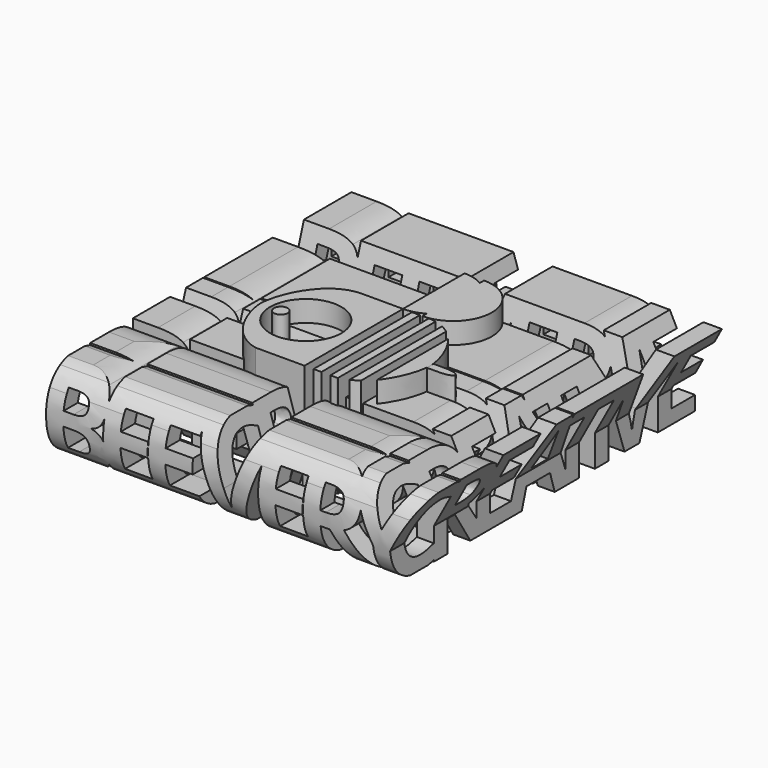
from build123d import *

# Parameters (mm, degrees)
F0_W     = 0.4192708333
F0_H     = 3.4461805556
F0_H_2   = 3.4722222222
F1_DEPTH = 200
F2_W     = 0.579117015
F2_H     = 3.4982638889
F3_DEPTH = 200
F6_DEPTH = 25
F5_W     = 1.9421083595
F5_H     = 30.1811452955
F5_R     = 8.7336650025
F5_R_2   = 1.6761545088


# Not quite as in the source:
# - a feature of the source that left no trace in its solid (it failed there, or was rolled back) is left out
# - a feature names something its author has since deleted; it is built from what else it names


with BuildPart() as f1:
    # F0 (on Front) → F1 (new body)
    with BuildSketch(Plane.XZ):
        with BuildLine():
            Line((8.6675347222, 19.8307291667), (2.4956597222, 19.8307291667))
            Line((2.4956597222, 19.8307291667), (2.4956597222, 0))
            Line((2.4956597222, 0), (9.9131944444, 0))
            add(Edge.make_bspline(
                [(15.2387152778, 1.5190972222), (13.2769097222, 0), (9.9131944444, 0)],
                knots=[0, 0, 0, 1, 1, 1], degree=2))
            add(Edge.make_bspline(
                [(16.4956597222, 2.9277045824), (16.024595477, 2.1276327747), (15.2387152778, 1.5190972222)],
                knots=[0.5994097392, 0.5994097392, 0.5994097392, 1, 1, 1], degree=2))
            Line((16.4956597222, 2.9277045824), (16.4956597222, 8.6243749651))
            add(Edge.make_bspline(
                [(16.3650173611, 8.8172743056), (16.4331135713, 8.7233545974), (16.4956597222, 8.6243749651)],
                knots=[0, 0, 0, 0.0815032043, 0.0815032043, 0.0815032043], degree=2))
            add(Edge.make_bspline(
                [(13.6458333333, 10.390625), (15.5295138889, 9.9696180556), (16.3650173611, 8.8172743056)],
                knots=[0, 0, 0, 1, 1, 1], degree=2))
            Line((13.6458333333, 10.390625), (13.6458333333, 10.5251736111))
            add(Edge.make_bspline(
                [(15.8637152778, 11.89453125), (15.0303819444, 10.7552083333), (13.6458333333, 10.5251736111)],
                knots=[0, 0, 0, 1, 1, 1], degree=2))
            add(Edge.make_bspline(
                [(16.4956597222, 13.2184769116), (16.2873852443, 12.4737675324), (15.8637152778, 11.89453125)],
                knots=[0.4915960401, 0.4915960401, 0.4915960401, 1, 1, 1], degree=2))
            Line((16.4956597222, 13.2184769116), (16.4956597222, 16.3653214947))
            add(Edge.make_bspline(
                [(14.7916666667, 18.6306423611), (16.0775950191, 17.8207125446), (16.4956597222, 16.3653214947)],
                knots=[0, 0, 0, 0.6748926934, 0.6748926934, 0.6748926934], degree=2))
            add(Edge.make_bspline(
                [(8.6675347222, 19.8307291667), (12.8862847222, 19.8307291667), (14.7916666667, 18.6306423611)],
                knots=[0, 0, 0, 1, 1, 1], degree=2))
        make_face()
        with BuildLine():
            Line((6.7013888889, 3.4722222222), (6.7013888889, 8.6414930556))
            Line((6.7013888889, 8.6414930556), (9.3055555556, 8.6414930556))
            add(Edge.make_bspline(
                [(12.8298611111, 6.171875), (12.8298611111, 8.6414930556), (9.3055555556, 8.6414930556)],
                knots=[0, 0, 0, 1, 1, 1], degree=2))
            add(Edge.make_bspline(
                [(12.0030381944, 4.1362847222), (12.8298611111, 4.8003472222), (12.8298611111, 6.171875)],
                knots=[0, 0, 0, 1, 1, 1], degree=2))
            add(Edge.make_bspline(
                [(9.4401041667, 3.4722222222), (11.1762152778, 3.4722222222), (12.0030381944, 4.1362847222)],
                knots=[0, 0, 0, 1, 1, 1], degree=2))
            Line((9.4401041667, 3.4722222222), (6.7013888889, 3.4722222222))
        make_face(mode=Mode.SUBTRACT)
        with BuildLine():
            Line((9.140625, 11.9748263889), (6.7013888889, 11.9748263889))
            Line((6.7013888889, 11.9748263889), (6.7013888889, 16.3845486111))
            Line((6.7013888889, 16.3845486111), (8.9105902778, 16.3845486111))
            add(Edge.make_bspline(
                [(11.5494791667, 15.8897569444), (10.7161458333, 16.3845486111), (8.9105902778, 16.3845486111)],
                knots=[0, 0, 0, 1, 1, 1], degree=2))
            add(Edge.make_bspline(
                [(12.3828125, 14.2534722222), (12.3828125, 15.3949652778), (11.5494791667, 15.8897569444)],
                knots=[0, 0, 0, 1, 1, 1], degree=2))
            add(Edge.make_bspline(
                [(11.6167534722, 12.5043402778), (12.3828125, 13.0338541667), (12.3828125, 14.2534722222)],
                knots=[0, 0, 0, 1, 1, 1], degree=2))
            add(Edge.make_bspline(
                [(9.140625, 11.9748263889), (10.8506944444, 11.9748263889), (11.6167534722, 12.5043402778)],
                knots=[0, 0, 0, 1, 1, 1], degree=2))
        make_face(mode=Mode.SUBTRACT)
        with BuildLine():
            Line((16.4956597222, 19.8307291667), (16.4956597222, 16.3653214947))
            add(Edge.make_bspline(
                [(16.4956597222, 16.3653214947), (16.6970486111, 15.6642348346), (16.6970486111, 14.8133680556)],
                knots=[0.6748926934, 0.6748926934, 0.6748926934, 1, 1, 1], degree=2))
            add(Edge.make_bspline(
                [(16.6970486111, 14.8133680556), (16.6970486111, 13.9385660744), (16.4956597222, 13.2184769116)],
                knots=[0, 0, 0, 0.4915960401, 0.4915960401, 0.4915960401], degree=2))
            Line((16.4956597222, 13.2184769116), (16.4956597222, 8.6243749651))
            add(Edge.make_bspline(
                [(16.4956597222, 8.6243749651), (17.2005208333, 7.5089283285), (17.2005208333, 5.7508680556)],
                knots=[0.0815032043, 0.0815032043, 0.0815032043, 1, 1, 1], degree=2))
            add(Edge.make_bspline(
                [(17.2005208333, 5.7508680556), (17.2005208333, 4.1248650739), (16.4956597222, 2.9277045824)],
                knots=[0, 0, 0, 0.5994097392, 0.5994097392, 0.5994097392], degree=2))
            Line((16.4956597222, 2.9277045824), (16.4956597222, 0))
            Line((16.4956597222, 0), (27.4956597222, 0))
            Line((27.4956597222, 0), (27.4956597222, 3.4722222222))
            Line((27.4956597222, 3.4722222222), (20.7013888889, 3.4722222222))
            Line((20.7013888889, 3.4722222222), (20.7013888889, 8.5850694444))
            Line((20.7013888889, 8.5850694444), (27.4157986111, 8.5850694444))
            Line((27.4157986111, 8.5850694444), (27.4157986111, 12.03125))
            Line((27.4157986111, 12.03125), (20.7013888889, 12.03125))
            Line((20.7013888889, 12.03125), (20.7013888889, 16.3845486111))
            Line((20.7013888889, 16.3845486111), (27.4956597222, 16.3845486111))
            Line((27.4956597222, 16.3845486111), (27.4956597222, 19.8307291667))
            Line((27.4956597222, 19.8307291667), (16.4956597222, 19.8307291667))
        make_face()
        with BuildLine():
            Line((16.4956597222, 8.6243749651), (16.4956597222, 2.9277045824))
            add(Edge.make_bspline(
                [(17.2005208333, 5.7508680556), (17.2005208333, 4.1248650739), (16.4956597222, 2.9277045824)],
                knots=[0, 0, 0, 0.5994097392, 0.5994097392, 0.5994097392], degree=2))
            add(Edge.make_bspline(
                [(16.4956597222, 8.6243749651), (17.2005208333, 7.5089283285), (17.2005208333, 5.7508680556)],
                knots=[0.0815032043, 0.0815032043, 0.0815032043, 1, 1, 1], degree=2))
        make_face()
        with BuildLine():
            add(Edge.make_bspline(
                [(16.4956597222, 16.3653214947), (16.6970486111, 15.6642348346), (16.6970486111, 14.8133680556)],
                knots=[0.6748926934, 0.6748926934, 0.6748926934, 1, 1, 1], degree=2))
            Line((16.4956597222, 16.3653214947), (16.4956597222, 13.2184769116))
            add(Edge.make_bspline(
                [(16.6970486111, 14.8133680556), (16.6970486111, 13.9385660744), (16.4956597222, 13.2184769116)],
                knots=[0, 0, 0, 0.4915960401, 0.4915960401, 0.4915960401], degree=2))
        make_face()
        Polygon((38, 19.8307291667), (27.9149305556, 19.8307291667), (27.9149305556, 16.3845486111), (27.4956597222, 16.3845486111), (27.4956597222, 3.4722222222), (27.9149305556, 3.4722222222), (27.9149305556, 0), (38.9149305556, 0), (38.9149305556, 3.4722222222), (31.7013888889, 3.4722222222), (31.7013888889, 8.5850694444), (38.4157986111, 8.5850694444), (38.4157986111, 12.03125), (31.7013888889, 12.03125), (31.7013888889, 16.3845486111), (38.9149305556, 16.3845486111), (38.9149305556, 17.13375), align=None)
        with Locations((27.7052951389, 18.1076388889)):
            Rectangle(F0_W, F0_H)
        with Locations((27.7052951389, 1.7361111111)):
            Rectangle(F0_W, F0_H_2)
        with BuildLine():
            Line((42.2447916667, 19.8307291667), (38.9149305556, 19.8307291667))
            Line((38.9149305556, 19.8307291667), (38.9149305556, 17.13375))
            Line((38.9149305556, 17.13375), (44.7274305556, 0))
            Line((44.7274305556, 0), (49.3107638889, 0))
            Line((49.3107638889, 0), (54.4956597222, 15.2542106005))
            Line((54.4956597222, 15.2542106005), (54.4956597222, 19.8307291667))
            Line((54.4956597222, 19.8307291667), (51.8064236111, 19.8307291667))
            Line((51.8064236111, 19.8307291667), (48.0520833333, 8.0295138889))
            add(Edge.make_bspline(
                [(47.0321180556, 3.6631944444), (47.1840277778, 4.9088541667), (48.0520833333, 8.0295138889)],
                knots=[0, 0, 0, 1, 1, 1], degree=2))
            add(Edge.make_bspline(
                [(46.6197916667, 5.5946180556), (46.9539930556, 4.2057291667), (47.0321180556, 3.6631944444)],
                knots=[0, 0, 0, 1, 1, 1], degree=2))
            add(Edge.make_bspline(
                [(45.9774305556, 8.0295138889), (46.2855902778, 6.9835069444), (46.6197916667, 5.5946180556)],
                knots=[0, 0, 0, 1, 1, 1], degree=2))
            Line((45.9774305556, 8.0295138889), (42.2447916667, 19.8307291667))
        make_face()
        Polygon((38.9149305556, 19.8307291667), (38, 19.8307291667), (38.9149305556, 17.13375), align=None)
        Polygon((54.4956597222, 19.8307291667), (54.4956597222, 15.2542106005), (56.0512152778, 19.8307291667), align=None)
        Polygon((56.0512152778, 19.8307291667), (54.4956597222, 15.2542106005), (54.4956597222, 0), (65.4956597222, 0), (65.4956597222, 3.4722222222), (58.7013888889, 3.4722222222), (58.7013888889, 8.5850694444), (65.4157986111, 8.5850694444), (65.4157986111, 12.03125), (58.7013888889, 12.03125), (58.7013888889, 16.3845486111), (65.4956597222, 16.3845486111), (65.4956597222, 19.8307291667), align=None)
        with Locations((65.7052951389, 18.1076388889)):
            Rectangle(F0_W, F0_H)
        with BuildLine():
            Line((71.2725694444, 19.8307291667), (65.9149305556, 19.8307291667))
            Line((65.9149305556, 19.8307291667), (65.9149305556, 16.3845486111))
            Line((65.9149305556, 16.3845486111), (65.4956597222, 16.3845486111))
            Line((65.4956597222, 16.3845486111), (65.4956597222, 3.4722222222))
            Line((65.4956597222, 3.4722222222), (65.9149305556, 3.4722222222))
            Line((65.9149305556, 3.4722222222), (65.9149305556, 0))
            Line((65.9149305556, 0), (69.7013888889, 0))
            Line((69.7013888889, 0), (69.7013888889, 7.6085069444))
            Line((69.7013888889, 7.6085069444), (71.9366319444, 7.6085069444))
            Line((71.9366319444, 7.6085069444), (76.671875, 0))
            Line((76.671875, 0), (81.3376736111, 0))
            add(Edge.make_bspline(
                [(75.5043402778, 8.6414930556), (79.9835069444, 1.953125), (81.3376736111, 0)],
                knots=[0, 0, 0, 1, 1, 1], degree=2))
            add(Edge.make_bspline(
                [(78.2322048611, 10.7769097222), (77.2708333333, 9.4140625), (75.5043402778, 8.6414930556)],
                knots=[0, 0, 0, 1, 1, 1], degree=2))
            add(Edge.make_bspline(
                [(79.1935757147, 13.8859595975), (79.1927713045, 12.138615651), (78.2322048611, 10.7769097222)],
                knots=[0.0008374332, 0.0008374332, 0.0008374332, 1, 1, 1], degree=2))
            Line((79.1935757147, 13.8859595975), (76.5480062099, 18.8106278972))
            add(Edge.make_bspline(
                [(71.2725694444, 19.8307291667), (74.640758574, 19.8307291667), (76.5480062099, 18.8106278972)],
                knots=[0, 0, 0, 0.8326510466, 0.8326510466, 0.8326510466], degree=2))
        make_face()
        with BuildLine():
            Line((71.0555555556, 11.0286458333), (69.7013888889, 11.0286458333))
            Line((69.7013888889, 11.0286458333), (69.7013888889, 16.3845486111))
            Line((69.7013888889, 16.3845486111), (70.9774305556, 16.3845486111))
            add(Edge.make_bspline(
                [(73.9787326389, 15.7877604167), (73.0086805556, 16.3845486111), (70.9774305556, 16.3845486111)],
                knots=[0, 0, 0, 1, 1, 1], degree=2))
            add(Edge.make_bspline(
                [(74.9487847222, 13.7803819444), (74.9487847222, 15.1909722222), (73.9787326389, 15.7877604167)],
                knots=[0, 0, 0, 1, 1, 1], degree=2))
            add(Edge.make_bspline(
                [(74.0004340278, 11.6927083333), (74.9487847222, 12.3567708333), (74.9487847222, 13.7803819444)],
                knots=[0, 0, 0, 1, 1, 1], degree=2))
            add(Edge.make_bspline(
                [(71.0555555556, 11.0286458333), (73.0520833333, 11.0286458333), (74.0004340278, 11.6927083333)],
                knots=[0, 0, 0, 1, 1, 1], degree=2))
        make_face(mode=Mode.SUBTRACT)
        with Locations((65.7052951389, 1.7361111111)):
            Rectangle(F0_W, F0_H_2)
        with BuildLine():
            add(Edge.make_bspline(
                [(76.5480062099, 18.8106278972), (76.9313311298, 18.6056045799), (77.2556423611, 18.359375)],
                knots=[0.8326510466, 0.8326510466, 0.8326510466, 1, 1, 1], degree=2))
            Line((76.5480062099, 18.8106278972), (79.1935757147, 13.8859595975))
            add(Edge.make_bspline(
                [(79.1935763889, 13.8888888889), (79.1935763889, 13.8874241078), (79.1935757147, 13.8859595975)],
                knots=[0, 0, 0, 0.0008374332, 0.0008374332, 0.0008374332], degree=2))
            add(Edge.make_bspline(
                [(77.2556423611, 18.359375), (79.1935763889, 16.8880208333), (79.1935763889, 13.8888888889)],
                knots=[0, 0, 0, 1, 1, 1], degree=2))
        make_face()
        with BuildLine():
            Line((76, 19.8307291667), (76.5480062099, 18.8106278972))
            add(Edge.make_bspline(
                [(76.5480062099, 18.8106278972), (76.9313311298, 18.6056045799), (77.2556423611, 18.359375)],
                knots=[0.8326510466, 0.8326510466, 0.8326510466, 1, 1, 1], degree=2))
            add(Edge.make_bspline(
                [(77.2556423611, 18.359375), (79.1935763889, 16.8880208333), (79.1935763889, 13.8888888889)],
                knots=[0, 0, 0, 1, 1, 1], degree=2))
            add(Edge.make_bspline(
                [(79.1935763889, 13.8888888889), (79.1935763889, 13.8874241078), (79.1935757147, 13.8859595975)],
                knots=[0, 0, 0, 0.0008374332, 0.0008374332, 0.0008374332], degree=2))
            Line((79.1935757147, 13.8859595975), (82.5798611111, 7.5824652778))
            Line((82.5798611111, 7.5824652778), (82.5798611111, 0))
            Line((82.5798611111, 0), (86.7552083333, 0))
            Line((86.7552083333, 0), (86.7552083333, 7.7170138889))
            Line((86.7552083333, 7.7170138889), (93.3350694444, 19.8307291667))
            Line((93.3350694444, 19.8307291667), (88.8038194444, 19.8307291667))
            Line((88.8038194444, 19.8307291667), (84.6675347222, 11.6666666667))
            Line((84.6675347222, 11.6666666667), (80.5572916667, 19.8307291667))
            Line((80.5572916667, 19.8307291667), (76, 19.8307291667))
        make_face()
    extrude(amount=-F1_DEPTH)


with BuildPart() as f3:
    # F2 (on Right) → F3 (new body)
    with BuildSketch(Plane.YZ):
        with BuildLine():
            add(Edge.make_bspline(
                [(10.9201388889, 16.6145833333), (8.5460069444, 16.6145833333), (7.2439236111, 14.8307291667)],
                knots=[0, 0, 0, 1, 1, 1], degree=2))
            add(Edge.make_bspline(
                [(13.1293402778, 16.2217881944), (12.0052083333, 16.6145833333), (10.9201388889, 16.6145833333)],
                knots=[0, 0, 0, 1, 1, 1], degree=2))
            add(Edge.make_bspline(
                [(15.1430216173, 15.405273706), (14.139687044, 15.8687519692), (13.1293402778, 16.2217881944)],
                knots=[0.1012204829, 0.1012204829, 0.1012204829, 1, 1, 1], degree=2))
            Line((15.1430216173, 15.405273706), (15.1430216173, 19.3729401919))
            add(Edge.make_bspline(
                [(10.9201388889, 20.1128472222), (13.023512731, 20.1128472222), (15.1430216173, 19.3729401919)],
                knots=[0, 0, 0, 0.7287478695, 0.7287478695, 0.7287478695], degree=2))
            add(Edge.make_bspline(
                [(5.9765625, 18.8736979167), (8.0859375, 20.1128472222), (10.9201388889, 20.1128472222)],
                knots=[0, 0, 0, 1, 1, 1], degree=2))
            add(Edge.make_bspline(
                [(2.7408854167, 15.3081597222), (3.8671875, 17.6345486111), (5.9765625, 18.8736979167)],
                knots=[0, 0, 0, 1, 1, 1], degree=2))
            add(Edge.make_bspline(
                [(1.6145833333, 9.8871527778), (1.6145833333, 12.9817708333), (2.7408854167, 15.3081597222)],
                knots=[0, 0, 0, 1, 1, 1], degree=2))
            add(Edge.make_bspline(
                [(3.90625, 2.3524305556), (1.6145833333, 4.9782986111), (1.6145833333, 9.8871527778)],
                knots=[0, 0, 0, 1, 1, 1], degree=2))
            add(Edge.make_bspline(
                [(10.5251736111, -0.2734375), (6.1979166667, -0.2734375), (3.90625, 2.3524305556)],
                knots=[0, 0, 0, 1, 1, 1], degree=2))
            add(Edge.make_bspline(
                [(15.1430216173, 0.4333476683), (13.0325989806, -0.2734375), (10.5251736111, -0.2734375)],
                knots=[0.1675636814, 0.1675636814, 0.1675636814, 1, 1, 1], degree=2))
            Line((15.1430216173, 0.4333476683), (15.1430216173, 3.9934341916))
            add(Edge.make_bspline(
                [(10.9201388889, 3.2291666667), (12.708358779, 3.2291666667), (15.1430216173, 3.9934341916)],
                knots=[0, 0, 0, 0.8565610451, 0.8565610451, 0.8565610451], degree=2))
            add(Edge.make_bspline(
                [(5.9418402778, 9.8611111111), (5.9418402778, 3.2291666667), (10.9201388889, 3.2291666667)],
                knots=[0, 0, 0, 1, 1, 1], degree=2))
            add(Edge.make_bspline(
                [(7.2439236111, 14.8307291667), (5.9418402778, 13.046875), (5.9418402778, 9.8611111111)],
                knots=[0, 0, 0, 1, 1, 1], degree=2))
        make_face()
        with BuildLine():
            Line((15.1430216173, 19.3729401919), (15.1430216173, 15.405273706))
            add(Edge.make_bspline(
                [(15.3689236111, 15.2994791667), (15.2560170829, 15.3530768182), (15.1430216173, 15.405273706)],
                knots=[0, 0, 0, 0.1012204829, 0.1012204829, 0.1012204829], degree=2))
            Line((15.3689236111, 15.2994791667), (16.7230902778, 18.7196180556))
            add(Edge.make_bspline(
                [(15.1430216173, 19.3729401919), (15.9319382305, 19.0975344353), (16.7230902778, 18.7196180556)],
                knots=[0.7287478695, 0.7287478695, 0.7287478695, 1, 1, 1], degree=2))
        make_face()
        with BuildLine():
            add(Edge.make_bspline(
                [(15.3689236111, 15.2994791667), (15.2560170829, 15.3530768182), (15.1430216173, 15.405273706)],
                knots=[0, 0, 0, 0.1012204829, 0.1012204829, 0.1012204829], degree=2))
            Line((15.1430216173, 15.405273706), (15.1430216173, 3.9934341916))
            add(Edge.make_bspline(
                [(15.1430216173, 3.9934341916), (15.5507281026, 4.1214177553), (15.9765625, 4.2708333333)],
                knots=[0.8565610451, 0.8565610451, 0.8565610451, 1, 1, 1], degree=2))
            Line((15.9765625, 4.2708333333), (15.9765625, 0.7465277778))
            add(Edge.make_bspline(
                [(15.9765625, 0.7465277778), (15.5678351175, 0.575618641), (15.1430216173, 0.4333476683)],
                knots=[0, 0, 0, 0.1675636814, 0.1675636814, 0.1675636814], degree=2))
            Line((15.1430216173, 0.4333476683), (15.1430216173, 0))
            Line((15.1430216173, 0), (19.348750784, 0))
            Line((19.348750784, 0), (19.348750784, 7.6085069444))
            Line((19.348750784, 7.6085069444), (21.5839938395, 7.6085069444))
            Line((21.5839938395, 7.6085069444), (26.3192368951, 0))
            Line((26.3192368951, 0), (28.2236685377, 0))
            Line((28.2236685377, 0), (28.2236685377, 4.0653140771))
            add(Edge.make_bspline(
                [(25.1517021728, 8.6414930556), (26.9354919994, 5.9779076654), (28.2236685377, 4.0653140771)],
                knots=[0, 0, 0, 0.3982414496, 0.3982414496, 0.3982414496], degree=2))
            add(Edge.make_bspline(
                [(27.8795667562, 10.7769097222), (26.9181952284, 9.4140625), (25.1517021728, 8.6414930556)],
                knots=[0, 0, 0, 1, 1, 1], degree=2))
            add(Edge.make_bspline(
                [(28.2236685377, 11.3337737786), (28.0705970875, 11.0477156998), (27.8795667562, 10.7769097222)],
                knots=[0.8012939579, 0.8012939579, 0.8012939579, 1, 1, 1], degree=2))
            Line((28.2236685377, 11.3337737786), (28.2236685377, 16.7875339058))
            add(Edge.make_bspline(
                [(26.9030042562, 18.359375), (27.7472161778, 17.7184167885), (28.2236685377, 16.7875339058)],
                knots=[0, 0, 0, 0.4356246959, 0.4356246959, 0.4356246959], degree=2))
            add(Edge.make_bspline(
                [(20.9199313395, 19.8307291667), (24.9650702284, 19.8307291667), (26.9030042562, 18.359375)],
                knots=[0, 0, 0, 1, 1, 1], degree=2))
            Line((20.9199313395, 19.8307291667), (15.1430216173, 19.8307291667))
            Line((15.1430216173, 19.8307291667), (15.1430216173, 19.3729401919))
            add(Edge.make_bspline(
                [(15.1430216173, 19.3729401919), (15.9319382305, 19.0975344353), (16.7230902778, 18.7196180556)],
                knots=[0.7287478695, 0.7287478695, 0.7287478695, 1, 1, 1], degree=2))
            Line((16.7230902778, 18.7196180556), (15.3689236111, 15.2994791667))
        make_face()
        with BuildLine():
            Line((20.7029174506, 11.0286458333), (19.348750784, 11.0286458333))
            Line((19.348750784, 11.0286458333), (19.348750784, 16.3845486111))
            Line((19.348750784, 16.3845486111), (20.6247924506, 16.3845486111))
            add(Edge.make_bspline(
                [(23.626094534, 15.7877604167), (22.6560424506, 16.3845486111), (20.6247924506, 16.3845486111)],
                knots=[0, 0, 0, 1, 1, 1], degree=2))
            add(Edge.make_bspline(
                [(24.5961466173, 13.7803819444), (24.5961466173, 15.1909722222), (23.626094534, 15.7877604167)],
                knots=[0, 0, 0, 1, 1, 1], degree=2))
            add(Edge.make_bspline(
                [(23.6477959228, 11.6927083333), (24.5961466173, 12.3567708333), (24.5961466173, 13.7803819444)],
                knots=[0, 0, 0, 1, 1, 1], degree=2))
            add(Edge.make_bspline(
                [(20.7029174506, 11.0286458333), (22.6994452284, 11.0286458333), (23.6477959228, 11.6927083333)],
                knots=[0, 0, 0, 1, 1, 1], degree=2))
        make_face(mode=Mode.SUBTRACT)
        with BuildLine():
            add(Edge.make_bspline(
                [(15.1430216173, 3.9934341916), (15.5507281026, 4.1214177553), (15.9765625, 4.2708333333)],
                knots=[0.8565610451, 0.8565610451, 0.8565610451, 1, 1, 1], degree=2))
            Line((15.1430216173, 3.9934341916), (15.1430216173, 0.4333476683))
            add(Edge.make_bspline(
                [(15.9765625, 0.7465277778), (15.5678351175, 0.575618641), (15.1430216173, 0.4333476683)],
                knots=[0, 0, 0, 0.1675636814, 0.1675636814, 0.1675636814], degree=2))
            Line((15.9765625, 0.7465277778), (15.9765625, 4.2708333333))
        make_face()
        with BuildLine():
            Line((28.2236685377, 19.8307291667), (28.2236685377, 16.7875339058))
            add(Edge.make_bspline(
                [(28.2236685377, 16.7875339058), (28.840938284, 15.5815248919), (28.840938284, 13.8888888889)],
                knots=[0.4356246959, 0.4356246959, 0.4356246959, 1, 1, 1], degree=2))
            add(Edge.make_bspline(
                [(28.840938284, 13.8888888889), (28.840938284, 12.4873200303), (28.2236685377, 11.3337737786)],
                knots=[0, 0, 0, 0.8012939579, 0.8012939579, 0.8012939579], degree=2))
            Line((28.2236685377, 11.3337737786), (28.2236685377, 4.0653140771))
            add(Edge.make_bspline(
                [(28.2236685377, 4.0653140771), (30.1701541359, 1.1753096687), (30.9850355062, 0)],
                knots=[0.3982414496, 0.3982414496, 0.3982414496, 1, 1, 1], degree=2))
            Line((30.9850355062, 0), (37.5626759736, 0))
            Line((37.5626759736, 0), (38.7834027488, 3.4722222222))
            Line((38.7834027488, 3.4722222222), (32.4293977044, 3.4722222222))
            Line((32.4293977044, 3.4722222222), (32.4293977044, 8.5850694444))
            Line((32.4293977044, 8.5850694444), (39.1438074266, 8.5850694444))
            Line((39.1438074266, 8.5850694444), (39.1438074266, 12.03125))
            Line((39.1438074266, 12.03125), (32.4293977044, 12.03125))
            Line((32.4293977044, 12.03125), (32.4293977044, 16.3845486111))
            Line((32.4293977044, 16.3845486111), (39.6429393711, 16.3845486111))
            Line((39.6429393711, 16.3845486111), (39.6429393711, 19.8307291667))
            Line((39.6429393711, 19.8307291667), (28.2236685377, 19.8307291667))
        make_face()
        with BuildLine():
            add(Edge.make_bspline(
                [(28.2236685377, 16.7875339058), (28.840938284, 15.5815248919), (28.840938284, 13.8888888889)],
                knots=[0.4356246959, 0.4356246959, 0.4356246959, 1, 1, 1], degree=2))
            Line((28.2236685377, 16.7875339058), (28.2236685377, 11.3337737786))
            add(Edge.make_bspline(
                [(28.840938284, 13.8888888889), (28.840938284, 12.4873200303), (28.2236685377, 11.3337737786)],
                knots=[0, 0, 0, 0.8012939579, 0.8012939579, 0.8012939579], degree=2))
        make_face()
        with BuildLine():
            add(Edge.make_bspline(
                [(28.2236685377, 4.0653140771), (30.1701541359, 1.1753096687), (30.9850355062, 0)],
                knots=[0.3982414496, 0.3982414496, 0.3982414496, 1, 1, 1], degree=2))
            Line((28.2236685377, 4.0653140771), (28.2236685377, 0))
            Line((28.2236685377, 0), (30.9850355062, 0))
        make_face()
        Polygon((38.7834027488, 3.4722222222), (37.5626759736, 0), (39.6429393711, 0), (39.6429393711, 3.4722222222), align=None)
        Polygon((39.6429393711, 3.4722222222), (39.6429393711, 0), (42.0939259736, 0), (43.5305579181, 4.7222222222), (50.7614606958, 4.7222222222), (52.1980926403, 0), (55.4927141121, 0), (55.4927141121, 3.5044173486), (50.9659901371, 16.3324652778), (50.1064293899, 16.3324652778), (50.1064293899, 18.7683298289), (49.7024329181, 19.9131944444), (44.5635440292, 19.9131944444), (38.7834027488, 3.4722222222), align=None)
        with BuildLine():
            add(Edge.make_bspline(
                [(49.7545162514, 8.2465277778), (47.7623287514, 14.6614583333), (47.5105926403, 15.5034722222)],
                knots=[0, 0, 0, 1, 1, 1], degree=2))
            Line((49.7545162514, 8.2465277778), (44.5895856958, 8.2465277778))
            add(Edge.make_bspline(
                [(47.1503495847, 16.8315972222), (46.7033009736, 15.0954861111), (44.5895856958, 8.2465277778)],
                knots=[0, 0, 0, 1, 1, 1], degree=2))
            add(Edge.make_bspline(
                [(47.5105926403, 15.5034722222), (47.2588565292, 16.3454861111), (47.1503495847, 16.8315972222)],
                knots=[0, 0, 0, 1, 1, 1], degree=2))
        make_face(mode=Mode.SUBTRACT)
        Polygon((50.1064293899, 19.8307291667), (50.1064293899, 18.7683298289), (50.9659901371, 16.3324652778), (55.4927141121, 16.3324652778), (55.4927141121, 3.5044173486), (56.7293426403, 0), (59.6984432788, 0), (59.6984432788, 16.3324652778), (64.5012707082, 16.3324652778), (64.5012707082, 19.8307291667), align=None)
        Polygon((50.9659901371, 16.3324652778), (50.1064293899, 18.7683298289), (50.1064293899, 16.3324652778), align=None)
        Polygon((55.4927141121, 3.5044173486), (55.4927141121, 0), (56.7293426403, 0), align=None)
        with Locations((64.7908292157, 18.0815972222)):
            Rectangle(F2_W, F2_H)
        Polygon((66.852924768, 19.8307291667), (65.0803877232, 19.8307291667), (65.0803877232, 16.3324652778), (64.5012707082, 16.3324652778), (64.5012707082, 0), (68.7069998749, 0), (68.7069998749, 14.3653942226), align=None)
        Polygon((68.7069998749, 19.8307291667), (66.852924768, 19.8307291667), (68.7069998749, 14.3653942226), align=None)
        with BuildLine():
            Line((71.0977164347, 19.8307291667), (68.7069998749, 19.8307291667))
            Line((68.7069998749, 19.8307291667), (68.7069998749, 14.3653942226))
            Line((68.7069998749, 14.3653942226), (73.5803553236, 0))
            Line((73.5803553236, 0), (78.1636886569, 0))
            Line((78.1636886569, 0), (83.796961459, 16.5733570077))
            Line((83.796961459, 16.5733570077), (83.796961459, 19.8307291667))
            Line((83.796961459, 19.8307291667), (80.6593483791, 19.8307291667))
            Line((80.6593483791, 19.8307291667), (76.9050081013, 8.0295138889))
            add(Edge.make_bspline(
                [(75.8850428236, 3.6631944444), (76.0369525458, 4.9088541667), (76.9050081013, 8.0295138889)],
                knots=[0, 0, 0, 1, 1, 1], degree=2))
            add(Edge.make_bspline(
                [(75.4727164347, 5.5946180556), (75.8069178236, 4.2057291667), (75.8850428236, 3.6631944444)],
                knots=[0, 0, 0, 1, 1, 1], degree=2))
            add(Edge.make_bspline(
                [(74.8303553236, 8.0295138889), (75.1385150458, 6.9835069444), (75.4727164347, 5.5946180556)],
                knots=[0, 0, 0, 1, 1, 1], degree=2))
            Line((74.8303553236, 8.0295138889), (71.0977164347, 19.8307291667))
        make_face()
        Polygon((83.796961459, 19.8307291667), (83.796961459, 16.5733570077), (84.9041400458, 19.8307291667), align=None)
        Polygon((84.9041400458, 19.8307291667), (83.796961459, 16.5733570077), (83.796961459, 0), (95.2162322924, 0), (95.2162322924, 3.4722222222), (88.0026906257, 3.4722222222), (88.0026906257, 8.5850694444), (94.7171003479, 8.5850694444), (94.7171003479, 12.03125), (88.0026906257, 12.03125), (88.0026906257, 16.3845486111), (95.2162322924, 16.3845486111), (95.2162322924, 19.8307291667), align=None)
    extrude(amount=F3_DEPTH)


with BuildPart() as f1_1:
    add(f1.part)

    # F4: intersect F3
    add(f3.part, mode=Mode.INTERSECT)


with BuildPart() as f6:
    # F5 (on Top) → F6 (new body)
    with BuildSketch(Plane.XY):
        with BuildLine():
            Line((46.6457828879, 74.7161057581), (46.6457828879, 55.8297485113))
            ThreePointArc((46.6457828879, 55.8297485113), (49.1214375344, 56.1600375499), (51.4239128679, 57.1277999775))
            Line((51.4239128679, 57.1277999774), (51.4239128679, 73.418054292))
            ThreePointArc((51.4239128679, 73.418054292), (49.1214375344, 74.3858167195), (46.6457828879, 74.7161057581))
        make_face()
        with BuildLine():
            ThreePointArc((51.4239128679, 73.418054292), (56.0889615113, 65.2729271347), (51.4239128679, 57.1277999775))
            Line((51.4239128679, 57.1277999774), (51.4239128679, 55.8297485113))
            ThreePointArc((51.4239128679, 55.8297485113), (60.8670914913, 65.2729271347), (51.4239128679, 74.7161057581))
            Line((51.4239128679, 74.7161057581), (51.4239128679, 73.418054292))
        make_face()
        with BuildLine():
            Line((51.4239128679, 73.418054292), (51.4239128679, 57.1277999774))
            ThreePointArc((51.4239128679, 57.1277999775), (56.0889615113, 65.2729271347), (51.4239128679, 73.418054292))
        make_face()
    extrude(amount=F6_DEPTH)


with BuildPart() as f6b:
    # F5 (on Top) → F6, piece 2 (new body)
    with BuildSketch(Plane.XY):
        with BuildLine():
            add(Edge.make_bspline(
                [(58.9525662363, 53.6522320745), (58.3473898746, 54.1146873914), (57.6987661118, 54.5195646008), (57.0061812435, 54.8507284851)],
                knots=[14.255985298, 14.255985298, 14.255985298, 14.255985298, 16.2148765473, 16.2148765473, 16.2148765473, 16.2148765473], degree=3))
            Line((57.0061812435, 54.8507284851), (57.0061812435, 26.4416613699))
            add(Edge.make_bspline(
                [(58.9525662363, 27.638332253), (58.3474475868, 27.1764418284), (57.6988317211, 26.772181434), (57.0061812435, 26.4416613699)],
                knots=[14.2772875072, 14.2772875072, 14.2772875072, 14.2772875072, 16.2352021693, 16.2352021693, 16.2352021693, 16.2352021693], degree=3))
            Line((58.9525662363, 27.638332253), (58.9525662363, 53.6522320745))
        make_face()
    extrude(amount=F6_DEPTH)


with BuildPart() as f6c:
    # F5 (on Top) → F6, piece 3 (new body)
    with BuildSketch(Plane.XY):
        with BuildLine():
            add(Edge.make_bspline(
                [(54.80453372, 55.6051160907), (54.2246879728, 55.7300830634), (53.6203089895, 55.8055179332), (52.9911862944, 55.8248097594)],
                knots=[18.166656566, 18.166656566, 18.166656566, 18.166656566, 19.621578867, 19.621578867, 19.621578867, 19.621578867], degree=3))
            Line((52.9911862944, 55.8248097594), (52.9911862944, 25.6486032158))
            Line((52.9911862944, 25.6486032158), (54.6046450428, 25.6486032158))
            add(Edge.make_bspline(
                [(54.80453372, 25.6893480965), (54.7382256115, 25.6751158197), (54.671596162, 25.6615309052), (54.6046450428, 25.6486032158)],
                knots=[18.1856427068, 18.1856427068, 18.1856427068, 18.1856427068, 18.3518904001, 18.3518904001, 18.3518904001, 18.3518904001], degree=3))
            Line((54.80453372, 25.6893480965), (54.80453372, 55.6051160907))
        make_face()
    extrude(amount=F6_DEPTH)


with BuildPart() as f6d:
    # F5 (on Top) → F6, piece 4 (new body)
    with BuildSketch(Plane.XY):
        with Locations((49.8184845911, 40.7391758636)):
            Rectangle(F5_W, F5_H)
    extrude(amount=F6_DEPTH)


with BuildPart() as f6e:
    # F5 (on Top) → F6, piece 5 (new body)
    with BuildSketch(Plane.XY):
        with BuildLine():
            Line((46.6457828879, 25.6486032158), (46.6457828879, 55.8297485113))
            Line((46.6457828879, 55.8297485113), (36.7094427347, 55.8297485113))
            add(Edge.make_bspline(
                [(23.9175353375, 40.6262278557), (23.9175353375, 45.149423182), (28.0028171837, 55.8297485113), (36.7094427347, 55.8297485113)],
                knots=[0, 0, 0, 0, 19.8690698117, 19.8690698117, 19.8690698117, 19.8690698117], degree=3))
            add(Edge.make_bspline(
                [(23.9175353375, 40.6262278557), (23.9238345748, 36.4770871086), (27.3755427315, 27.1522740315), (34.6666945628, 25.6486032158)],
                knots=[0, 0, 0, 0, 18.2259788101, 18.2259788101, 18.2259788101, 18.2259788101], degree=3))
            Line((34.6666945628, 25.6486032158), (46.6457828879, 25.6486032158))
        make_face()
        with Locations((34.9984728904, 40.5927539753)):
            Circle(F5_R, mode=Mode.SUBTRACT)
    extrude(amount=F6_DEPTH)


with BuildPart() as f6f:
    # F5 (on Top) → F6, piece 6 (new body)
    with BuildSketch(Plane.XY):
        with Locations((28.8337614649, 40.6571228374)):
            Circle(F5_R_2)
    extrude(amount=F6_DEPTH)


with BuildPart() as f6g:
    # F5 (on Top) → F6, piece 7 (new body)
    with BuildSketch(Plane.XY):
        with BuildLine():
            Line((65.4598921537, 41.6880458391), (65.4598921537, 40.6892975067))
            Line((65.4598921537, 40.6892975067), (65.4598921537, 40.6262278557))
            Line((65.4598921537, 40.6262278557), (65.4598921537, 39.6274977335))
            add(Edge.make_bspline(
                [(65.4598921537, 39.6274977335), (68.2962250362, 39.5967156875), (71.0435203604, 39.4597946758), (71.7080413799, 40.6625056756)],
                knots=[0.6398542104, 0.6398542104, 0.6398542104, 0.6398542104, 7.1161808092, 7.1161808092, 7.1161808092, 7.1161808092], degree=3))
            add(Edge.make_bspline(
                [(65.4598921537, 41.6880458391), (68.2956207924, 41.7231664397), (71.0418176618, 41.8639855073), (71.7080413799, 40.6625056756)],
                knots=[0.6410447359, 0.6410447359, 0.6410447359, 0.6410447359, 7.1161808092, 7.1161808092, 7.1161808092, 7.1161808092], degree=3))
        make_face()
    extrude(amount=F6_DEPTH)


with BuildPart() as f6h:
    # F5 (on Top) → F6, piece 8 (new body)
    with BuildSketch(Plane.XY):
        with BuildLine():
            add(Edge.make_bspline(
                [(65.3967591903, 41.6872821553), (65.0946221422, 44.4192907804), (63.7046510491, 48.4572601615), (61.1542137597, 51.51984798)],
                knots=[1.4238178437, 1.4238178437, 1.4238178437, 1.4238178437, 11.6288772148, 11.6288772148, 11.6288772148, 11.6288772148], degree=3))
            Line((61.1542137597, 51.51984798), (61.1542137597, 29.7693166623))
            add(Edge.make_bspline(
                [(65.3983222806, 39.6281485814), (65.0996903312, 36.8897884039), (63.7105172426, 32.8381683215), (61.1542137597, 29.7693166623)],
                knots=[1.4238178437, 1.4238178437, 1.4238178437, 1.4238178437, 11.6508972622, 11.6508972622, 11.6508972622, 11.6508972622], degree=3))
            add(Edge.make_bspline(
                [(65.459826372, 40.6577626494), (65.4589928071, 40.3421354551), (65.4385538655, 39.9970594434), (65.3983222806, 39.6281485814)],
                knots=[0.046029518, 0.046029518, 0.046029518, 0.046029518, 1.4238178437, 1.4238178437, 1.4238178437, 1.4238178437], degree=3))
            add(Edge.make_bspline(
                [(65.459826372, 40.6577626494), (65.4585136225, 40.9733882145), (65.4375508097, 41.3184327981), (65.3967591903, 41.6872821553)],
                knots=[0.046029518, 0.046029518, 0.046029518, 0.046029518, 1.4238178437, 1.4238178437, 1.4238178437, 1.4238178437], degree=3))
        make_face()
    extrude(amount=F6_DEPTH)


solid = Compound([f1_1.part, f6.part, f6b.part, f6c.part, f6d.part, f6e.part, f6f.part, f6g.part, f6h.part])
